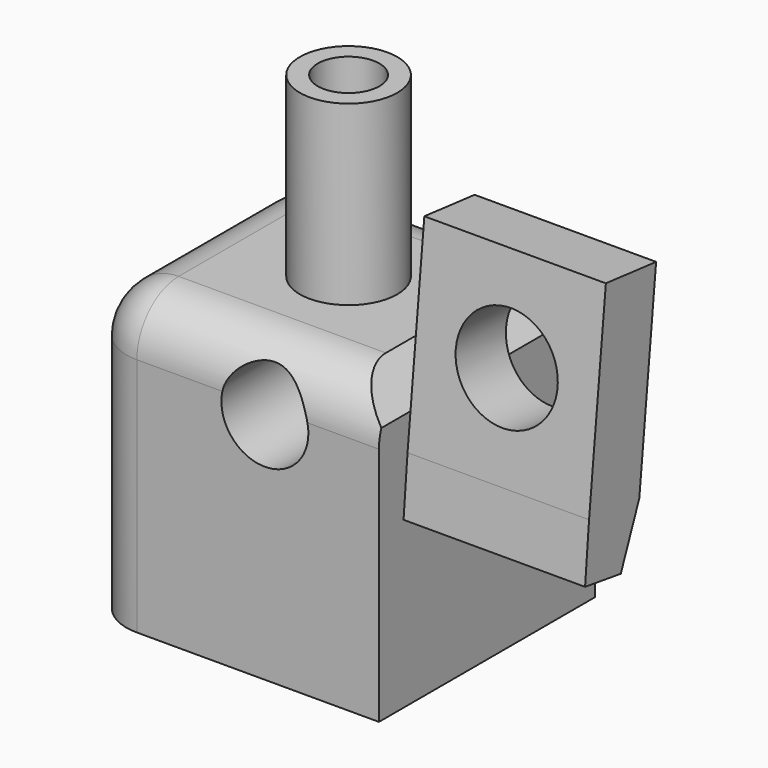
from build123d import *

# Parameters (mm, degrees)
F0_W           = 42.9559741169
F0_H           = 39.4349899143
F1_DEPTH       = 42.672
F3_D           = 12.7
F3_DEPTH       = 50.8
F3_TIP         = 3.8154649308
F5_D           = 12.7
F5_CBORE_D     = 15.24
F5_CBORE_DEPTH = 19.05
F6_SIZE        = 5.08
F7_T1_DEPTH    = 54.102
F7_T3_DEPTH    = 49.3059741169
F7_T5_DEPTH    = 24.1949899143
F7_S9_W        = 7.62
F7_S9_H        = 7.62
F7_T10_DEPTH   = 7.62
F7_S15_W       = 7.62
F7_S15_H       = 7.62
F7_T16_DEPTH   = 7.62
F11_R          = 7.1053142902
F12_DEPTH      = 25.9
F14_DEPTH      = 26.5
F15_DEPTH      = 29.3
F16_R          = 4.5
F17_DEPTH      = 25
F18_R          = 7.4357269109
F19_DEPTH      = 25


# Not quite as in the source:
# - a fillet or chamfer that OpenCascade refuses, or shapes differently, is made with other operations: its cross-section is extruded or revolved along the edge and cut away or added
# - the program builds the solid bodies; features that only make, move or delete a surface that nothing else refers to are left out


with BuildPart() as f1:
    # F0 (on Top) → F1 (new body)
    with BuildSketch(Plane.XY):
        with Locations((2.8086053208, -1.5343176201)):
            Rectangle(F0_W, F0_H)
    extrude(amount=F1_DEPTH)

    # F3
    with Locations(Plane.YZ.offset(24.2865923792)):
        with Locations((0, 21.336)):
            Hole(F3_D / 2, depth=F3_DEPTH)
            with Locations((0, 0, -(F3_DEPTH + F3_TIP / 2))):  # 118° drill point
                Cone(0, F3_D / 2, F3_TIP, mode=Mode.SUBTRACT)

    # F5 (through all)
    with Locations(Plane(origin=(0, 18.1831773371, 0), x_dir=(-1, 0, 0), z_dir=(0, 1, 0))):
        with Locations((-7.6360311359, 33.7194018066)):
            CounterBoreHole(F5_D / 2, F5_CBORE_D / 2, F5_CBORE_DEPTH)

    # F6
    f6_edges = [f1.edges().sort_by_distance(p)[0] for p in [
        (24.286592, -1.534318, 42.672),
    ]]
    chamfer(f6_edges, length=F6_SIZE)

    # F7: fillet of radius 7.62 on 5 edges, made by hand

    # F7_s2 → F7_t1 (cut)
    with BuildSketch(Plane.XY.offset(-19.05)):
        with BuildLine():
            ThreePointArc((-11.0493817377, 18.1831773371), (-16.4375354104, 15.9513310097), (-18.6693817377, 10.5631773371))
            Line((-18.6693817377, 10.5631773371), (-18.6693817377, 18.1831773371))
            Line((-18.6693817377, 18.1831773371), (-11.0493817377, 18.1831773371))
        make_face()
        with BuildLine():
            ThreePointArc((-18.6693817377, -13.6318125772), (-16.4375354104, -19.0199662499), (-11.0493817377, -21.2518125772))
            Line((-11.0493817377, -21.2518125772), (-18.6693817377, -21.2518125772))
            Line((-18.6693817377, -21.2518125772), (-18.6693817377, -13.6318125772))
        make_face()
    extrude(amount=F7_T1_DEPTH, mode=Mode.SUBTRACT)

    # F7_s4 → F7_t3 (cut)
    with BuildSketch(Plane.YZ.offset(-11.0493817377)):
        with BuildLine():
            ThreePointArc((18.1831773371, 35.052), (15.9513310097, 40.4401536726), (10.5631773371, 42.672))
            Line((10.5631773371, 42.672), (18.1831773371, 42.672))
            Line((18.1831773371, 42.672), (18.1831773371, 35.052))
        make_face()
        with BuildLine():
            ThreePointArc((-13.6318125772, 42.672), (-19.0199662499, 40.4401536726), (-21.2518125772, 35.052))
            Line((-21.2518125772, 35.052), (-21.2518125772, 42.672))
            Line((-21.2518125772, 42.672), (-13.6318125772, 42.672))
        make_face()
    extrude(amount=F7_T3_DEPTH, mode=Mode.SUBTRACT)

    # F7_s6 → F7_t5 (cut)
    with BuildSketch(Plane.XZ.offset(-10.5631773371)):
        with BuildLine():
            ThreePointArc((-11.0493817377, 42.672), (-16.4375354104, 40.4401536726), (-18.6693817377, 35.052))
            Line((-18.6693817377, 35.052), (-18.6693817377, 42.672))
            Line((-18.6693817377, 42.672), (-11.0493817377, 42.672))
        make_face()
    extrude(amount=F7_T5_DEPTH, mode=Mode.SUBTRACT)


with BuildPart() as f7_tool8:
    # F7_s9 → F7_t10 (new body)
    with BuildSketch(Plane.XZ.offset(-10.5631773371)):
        with Locations((-14.8593817377, 38.862)):
            Rectangle(F7_S9_W, F7_S9_H)
    extrude(amount=-F7_T10_DEPTH)

    # F7_s11 → F7_t12 (revolve, cut)
    with BuildSketch(Plane(origin=(-11.0493817377, 10.5631773371, 35.052), x_dir=(0.7071067812, 0, -0.7071067812), z_dir=(0.7071067812, 0, 0.7071067812))):
        with BuildLine():
            ThreePointArc((0, -7.62), (7.62, 0), (0, 7.62))
            Line((0, 7.62), (0, -7.62))
        make_face()
    revolve(axis=Axis((-11.0493817377, 10.5631773371, 35.052), (0, 1, 0)), mode=Mode.SUBTRACT)


with BuildPart() as f1_1:
    add(f1.part)

    # F7_t7: cut F7_tool8
    add(f7_tool8.part, mode=Mode.SUBTRACT)


with BuildPart() as f7_tool14:
    # F7_s15 → F7_t16 (new body)
    with BuildSketch(Plane.XY.offset(35.052)):
        with Locations((-14.8593817377, -17.4418125772)):
            Rectangle(F7_S15_W, F7_S15_H)
    extrude(amount=F7_T16_DEPTH)

    # F7_s17 → F7_t18 (revolve, cut)
    with BuildSketch(Plane(origin=(-11.0493817377, -13.6318125772, 35.052), x_dir=(0.7071067812, 0.7071067812, 0), z_dir=(0.7071067812, -0.7071067812, 0))):
        with BuildLine():
            ThreePointArc((0, -7.62), (7.62, 0), (0, 7.62))
            Line((0, 7.62), (0, -7.62))
        make_face()
    revolve(axis=Axis((-11.0493817377, -13.6318125772, 35.052), (0, 0, 1)), mode=Mode.SUBTRACT)


with BuildPart() as f1_2:
    add(f1_1.part)

    # F7_t13: cut F7_tool14
    add(f7_tool14.part, mode=Mode.SUBTRACT)

    # F11 (on face) → F12 (join)
    with BuildSketch(Plane.XY.offset(42.672)):
        with Locations((4.0786053208, -1.5343176201)):
            Circle(F11_R)
    extrude(amount=F12_DEPTH)

    # F13 (on face) → F14 (join)
    with BuildSketch(Plane.YZ.offset(24.2865923792)):
        Polygon((-6.8631088361, 31.5118990839), (-16.0354040563, 32.4774049222), (-16.7595334351, 24.1499263793), (-10.2423755452, 23.1844205409), align=None)
    extrude(amount=F14_DEPTH)

    # F15 (add): a face of the model
    f15_faces = [f1_2.faces().sort_by_distance(p)[0] for p in [
        (37.5365923792, -11.4492564462, 31.994652003),
    ]]
    extrude(f15_faces, amount=F15_DEPTH)

    # F16 (on face) → F17 (cut)
    with BuildSketch(Plane.XY.offset(68.572)):
        with Locations((4.0786053208, -1.5343176201)):
            Circle(F16_R)
    extrude(amount=-F17_DEPTH, mode=Mode.SUBTRACT)

    # F18 (on face) → F19 (cut)
    with BuildSketch(Plane(origin=(0, -10.0685909657, 1.0598528644), x_dir=(-1, 0, 0), z_dir=(0, 0.9945054407, -0.1046849002))):
        with Locations((-37.5365923792, 45.2702912239)):
            Circle(F18_R)
    extrude(amount=-F19_DEPTH, mode=Mode.SUBTRACT)


solid = f1_2.part
